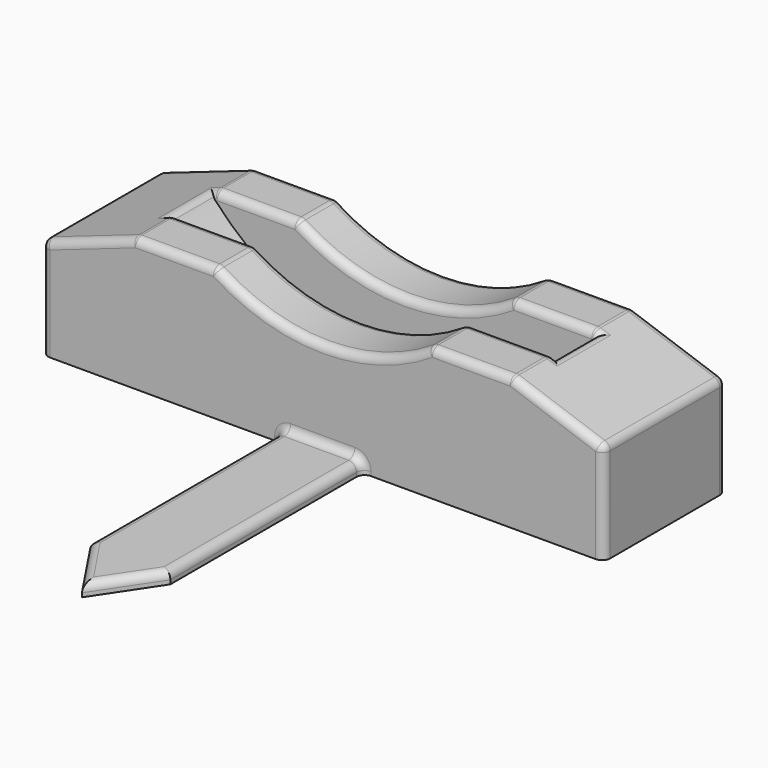
from build123d import *

# Parameters (mm, degrees)
F1_DEPTH  = 19.05
F2_R      = 63.5
F3_DEPTH  = 6.35
F4_R      = 2
F5_R      = 1.5
F6_DEPTH  = 33.001
F7_R      = 3
F8_DEPTH  = 7
F9_W      = 20
F9_H      = 3
F10_DEPTH = 75
F12_DEPTH = 3.001
F13_F1_R  = 2
F13_F2_R  = 2


with BuildPart() as f1:
    # F0 (on Front) → F1 (new body, symmetric)
    with BuildSketch(Plane.XZ):
        with BuildLine():
            Line((-70, -13), (70, -13))
            Line((70, -13), (70, 12))
            Line((70, 12), (47, 20))
            Line((47, 20), (26.6833281283, 20))
            ThreePointArc((26.6833281283, 20), (0, 12), (-26.6833281283, 20))
            Line((-26.6833281283, 20), (-47, 20))
            Line((-47, 20), (-70, 12))
            Line((-70, 12), (-70, -13))
        make_face()
    extrude(amount=F1_DEPTH, both=True)

    # F2 (on Front) → F3 (cut, symmetric)
    with BuildSketch(Plane.XZ):
        with Locations((0, 60.5)):
            Circle(F2_R)
    extrude(amount=F3_DEPTH, both=True, mode=Mode.SUBTRACT)

    # F4
    f4_edges = [f1.edges().sort_by_distance(p)[0] for p in [
        (-70, -19.05, -0.5),
        (-58.5, -19.05, 16),
        (-36.841664, -19.05, 20),
        (0, -19.05, 12),
        (36.841664, -19.05, 20),
        (58.5, -19.05, 16),
        (70, -19.05, -0.5),
        (70, 0, 12),
        (47, -12.7, 20),
        (26.683328, -12.7, 20),
        (26.683328, 12.7, 20),
        (47.738913, -6.35, 19.742987),
        (48.477826, 0, 19.485974),
        (47.738913, 6.35, 19.742987),
        (47, 12.7, 20),
        (58.5, 19.05, 16),
        (70, 19.05, -0.5),
        (0, 6.35, 12),
        (-26.683328, 12.7, 20),
        (0, 19.05, 12),
        (-26.683328, -12.7, 20),
        (0, -6.35, 12),
        (-47, -12.7, 20),
        (-36.841664, -6.35, 20),
        (-36.841664, 6.35, 20),
        (-47, 12.7, 20),
        (-36.841664, 19.05, 20),
        (-47.738913, 6.35, 19.742987),
        (-48.477826, 0, 19.485974),
        (-47.738913, -6.35, 19.742987),
        (-70, 0, 12),
        (-58.5, 19.05, 16),
        (-70, 19.05, -0.5),
        (36.841664, 6.35, 20),
        (36.841664, 19.05, 20),
        (36.841664, -6.35, 20),
    ]]
    fillet(f4_edges, radius=F4_R)

    # F5 (on face) → F6 (cut, through all)
    with BuildSketch(Plane(origin=(0, 0, -13), x_dir=(1, 0, 0), z_dir=(0, 0, -1))):
        Circle(F5_R)
    extrude(amount=-F6_DEPTH, mode=Mode.SUBTRACT)

    # F7 (on Top) → F8 (cut)
    with BuildSketch(Plane.XY):
        Circle(F7_R)
    extrude(amount=-F8_DEPTH, mode=Mode.SUBTRACT)

    # F9 (on face) → F10 (join)
    with BuildSketch(Plane.XZ.offset(19.05)):
        with Locations((0, -11.5)):
            Rectangle(F9_W, F9_H)
    extrude(amount=F10_DEPTH)

    # F11 (on face) → F12 (cut, through all)
    with BuildSketch(Plane.XY.offset(-10)):
        Polygon((-10, -94.05), (0, -94.05), (-10, -79.05), align=None)
        Polygon((10, -79.05), (0, -94.05), (10, -94.05), align=None)
    extrude(amount=-F12_DEPTH, mode=Mode.SUBTRACT)

    # F13: fillet of radius 2 on 5 edges, made by hand

    # F13_f1
    f13_f1_edges = [f1.edges().sort_by_distance(p)[0] for p in [
        (-10, -49.05, -10),
        (-5, -86.55, -10),
        (5, -86.55, -10),
        (10, -49.05, -10),
    ]]
    fillet(f13_f1_edges, radius=F13_F1_R)

    # F13_f2
    f13_f2_edges = [f1.edges().sort_by_distance(p)[0] for p in [
        (0, -19.05, -10),
        (9.4142135624, -19.05, -10.5857864376),
        (-9.4142135624, -19.05, -10.5857864376),
    ]]
    fillet(f13_f2_edges, radius=F13_F2_R)


solid = f1.part
